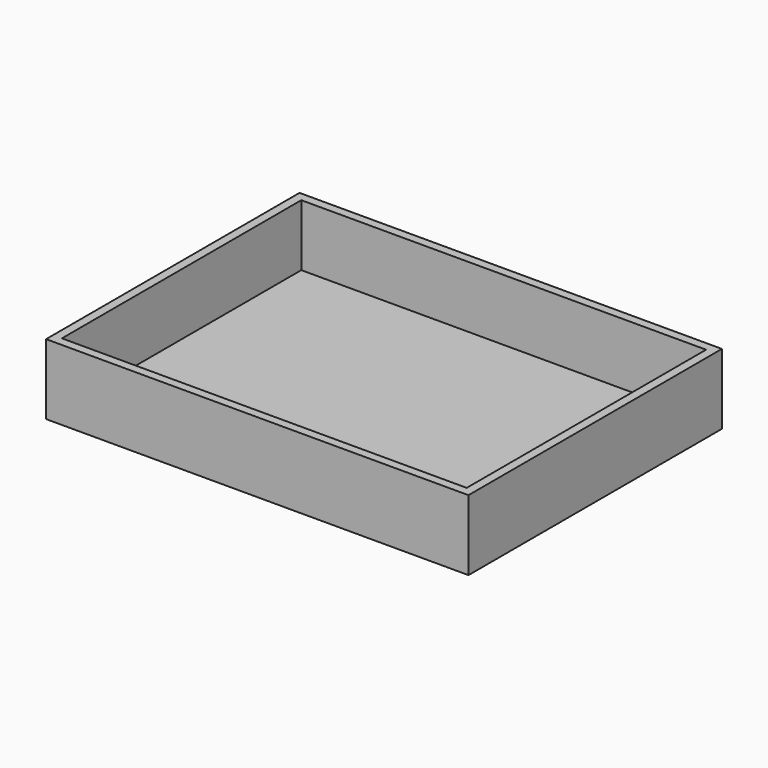
from build123d import *

# Parameters (mm, degrees)
F0_W     = 120
F0_H     = 90
F1_DEPTH = 20
F2_T     = -2.5


# Not quite as in the source:
# - a feature names something its author has since deleted; it is built from what else it names


with BuildPart() as f1:
    # F0 (on Top) → F1 (new body)
    with BuildSketch(Plane.XY):
        with Locations((0.2172155073, -0.1426615352)):
            Rectangle(F0_W, F0_H)
    extrude(amount=F1_DEPTH)

    # F2
    f2_openings = [f1.faces().sort_by_distance(p)[0] for p in [
        (0.217216, -0.142662, 20),
    ]]
    offset(amount=F2_T, openings=f2_openings)


solid = f1.part
